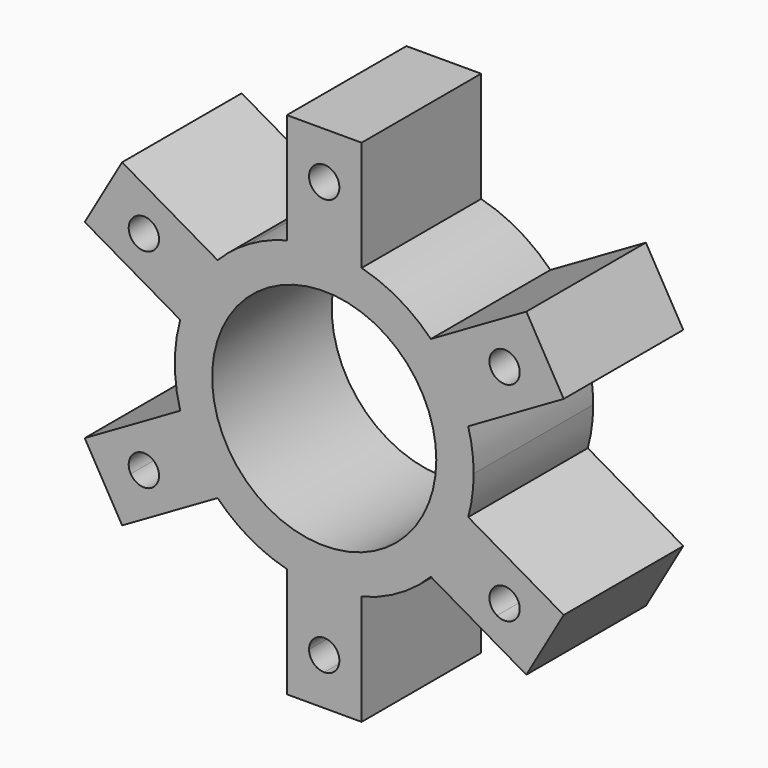
from build123d import *

# Parameters (mm, degrees)
F0_R            = 38.1
F1_DEPTH        = 25.4
F1_COPIES_COUNT = 6


# Not quite as in the source:
# - a feature of the source that left no trace in its solid (it failed there, or was rolled back) is left out
# - a pattern or mirror of a feature is missing from the dataset's text; its kind, count and spacing are read off the source's solid


with BuildPart() as f1:
    # F0 (on Front) → F1 (new body, symmetric)
    with BuildSketch(Plane.XZ):
        with BuildLine():
            ThreePointArc((-12.7, 49.1868884968), (-31.1085197333, -40.1609262841), (50.8, 0))
            ThreePointArc((50.8, 0), (40.1609262841, 31.1085197333), (12.7, 49.1868884968))
            ThreePointArc((12.7, 49.1868884968), (0, 50.8), (-12.7, 49.1868884968))
        make_face()
        Circle(F0_R, mode=Mode.SUBTRACT)
        with BuildLine():
            ThreePointArc((-12.7, 49.1868884968), (0, 50.8), (12.7, 49.1868884968))
            Line((12.7, 49.1868884968), (12.7, 86.6675451398))
            Line((12.7, 86.6675451398), (0, 86.6675451398))
            Line((0, 86.6675451398), (-12.7, 86.6675451398))
            Line((-12.7, 86.6675451398), (-12.7, 49.1868884968))
        make_face()
        with BuildLine():
            ThreePointArc((5.1527655949, 70.7925451398), (-3.643555494, 67.1489896457), (0, 75.9453107347))
            ThreePointArc((0, 75.9453107347), (3.643555494, 74.4361006338), (5.1527655949, 70.7925451398))
        make_face(mode=Mode.SUBTRACT)
    extrude(amount=F1_DEPTH, both=True)

    # F1_copies: F1 ×6 about axis
    f1_copies_axis = Axis((0, 0, 0), (0, 1, 0))


with BuildPart() as f1_1:
    add(f1.part)
    for i in range(1, F1_COPIES_COUNT):
        add(f1.part.rotate(f1_copies_axis, i * 360 / F1_COPIES_COUNT))


solid = f1_1.part
